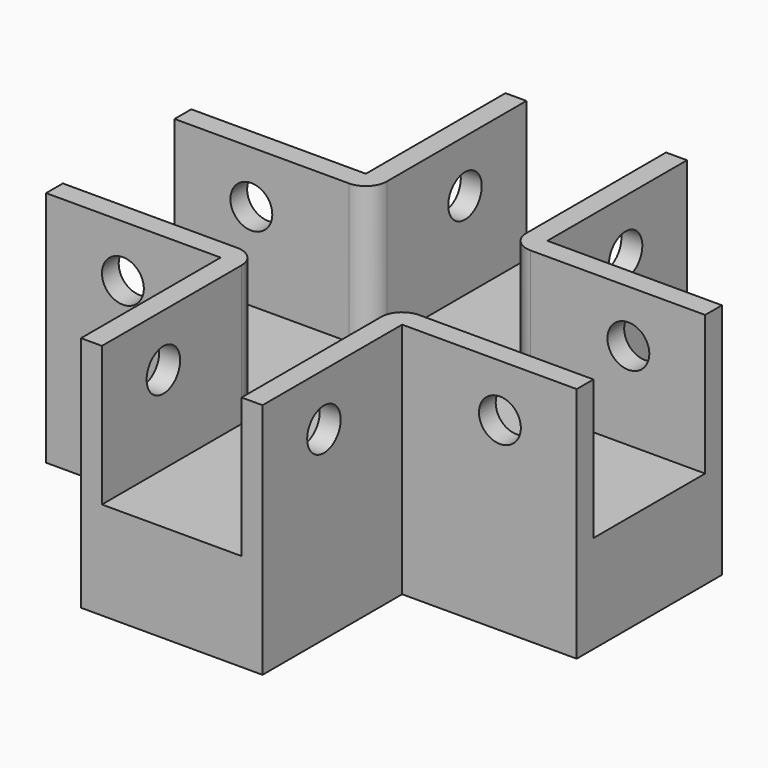
from build123d import *

# Parameters (mm, degrees)
F3_DEPTH              = 14
F5_DEPTH              = 20
F5_COPIES_COUNT       = 4
F8_D                  = 6
F8_DEPTH              = 3
F8_TIP                = 1.8025818571
F8_ON_F6_D            = 6
F8_ON_F6_DEPTH        = 3
F8_ON_F6_TIP          = 1.8025818571
F8_COPIES_COUNT       = 4
F8_ON_F6_COPIES_COUNT = 4
F9_R                  = 3


# Not quite as in the source:
# - a pattern or mirror of a feature is missing from the dataset's text; its kind, count and spacing are read off the source's solid


with BuildPart() as f3:
    # F2 (on Top) → F3 (new body)
    with BuildSketch(Plane.XY):
        Polygon((-13, 38), (-13, 13), (-38, 13), (-38, -13), (-13, -13), (-13, -38), (13, -38), (13, -13), (38, -13), (38, 13), (13, 13), (13, 38), align=None)
    extrude(amount=-F3_DEPTH)

    # F4 (on Top) → F5 (join)
    with BuildSketch(Plane.XY):
        Polygon((13, 38), (10, 38), (10, 10), (38, 10), (38, 13), (13, 13), align=None)
    f5 = extrude(amount=F5_DEPTH)

    # F5_copies: F5 ×4 about axis
    f5_copies_axis = Axis((0, 0, 0), (0, 0, 1))
    for i in range(1, F5_COPIES_COUNT):
        add(f5.rotate(f5_copies_axis, i * 360 / F5_COPIES_COUNT))

    # F8
    with Locations(Plane.YZ.offset(13)):
        with Locations((27, 12.5)):
            f8 = Hole(F8_D / 2, depth=F8_DEPTH)
            with Locations((0, 0, -(F8_DEPTH + F8_TIP / 2))):  # 118° drill point
                Cone(0, F8_D / 2, F8_TIP, mode=Mode.SUBTRACT)

    # F8 on F6
    with Locations(Plane(origin=(0, 13, 0), x_dir=(-1, 0, 0), z_dir=(0, 1, 0))):
        with Locations((-27, 12.5)):
            f8_on_f6 = Hole(F8_ON_F6_D / 2, depth=F8_ON_F6_DEPTH)
            with Locations((0, 0, -(F8_ON_F6_DEPTH + F8_ON_F6_TIP / 2))):  # 118° drill point
                Cone(0, F8_ON_F6_D / 2, F8_ON_F6_TIP, mode=Mode.SUBTRACT)

    # F8_copies: F8 ×4 about axis
    f8_copies_axis = Axis((0, 0, 0), (0, 0, 1))
    for i in range(1, F8_COPIES_COUNT):
        add(f8.rotate(f8_copies_axis, i * 360 / F8_COPIES_COUNT), mode=Mode.SUBTRACT)

    # F8 on F6_copies: F8 on F6 ×4 about axis
    f8_on_f6_copies_axis = Axis((0, 0, 0), (0, 0, 1))
    for i in range(1, F8_ON_F6_COPIES_COUNT):
        add(f8_on_f6.rotate(f8_on_f6_copies_axis, i * 360 / F8_ON_F6_COPIES_COUNT), mode=Mode.SUBTRACT)

    # F9
    f9_edges = [f3.edges().sort_by_distance(p)[0] for p in [
        (10, 10, 10),
        (-10, 10, 10),
        (-10, -10, 10),
        (10, -10, 10),
    ]]
    fillet(f9_edges, radius=F9_R)


solid = f3.part
